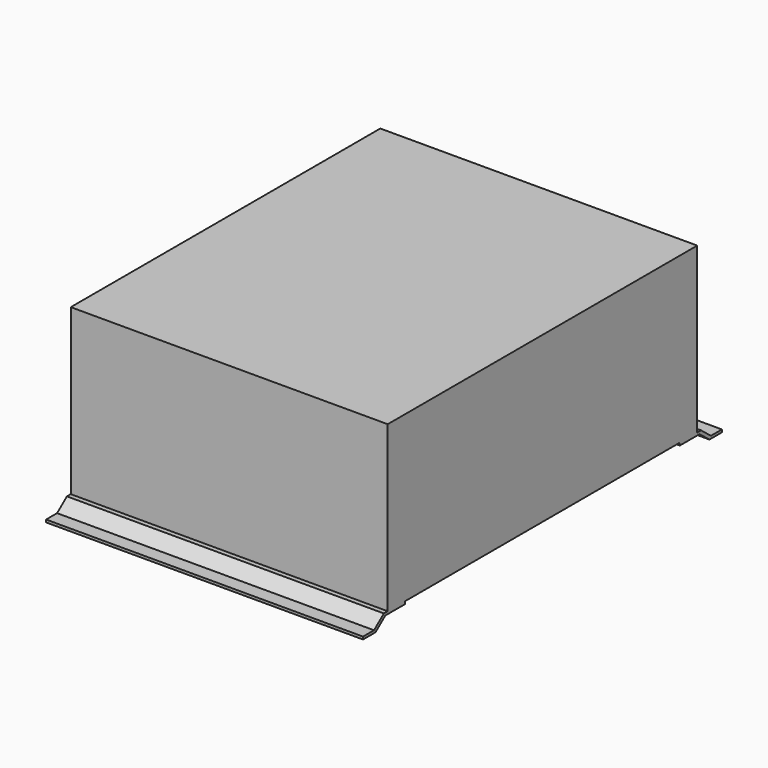
from build123d import *

# Parameters (mm, degrees)
F0_W     = 195.58
F0_H     = 238.76
F1_DEPTH = 101.6
F3_DEPTH = 195.58


# Not quite as in the source:
# - a pattern or mirror of a feature is missing from the dataset's text; its kind, count and spacing are read off the source's solid


with BuildPart() as f1:
    # F0 (on Top) → F1 (new body)
    with BuildSketch(Plane.XY):
        Rectangle(F0_W, F0_H)
    extrude(amount=F1_DEPTH)

    # F2 (on face) → F3 (join)
    with BuildSketch(Plane(origin=(-97.79, 0, 0), x_dir=(0, -1, 0), z_dir=(-1, 0, 0))):
        Polygon((122.3456934094, 0), (105.8921615149, 0), (105.8921615149, -1.5875), (121.2054859035, -1.5875), (128.7959814072, -7.62), (138.43, -7.62), (138.43, -6.0325), (129.9361889131, -6.0325), align=None)
    f3 = extrude(amount=-F3_DEPTH)

    # F3_copies: F3 across plane
    add(f3.mirror(Plane.ZX))


solid = f1.part
